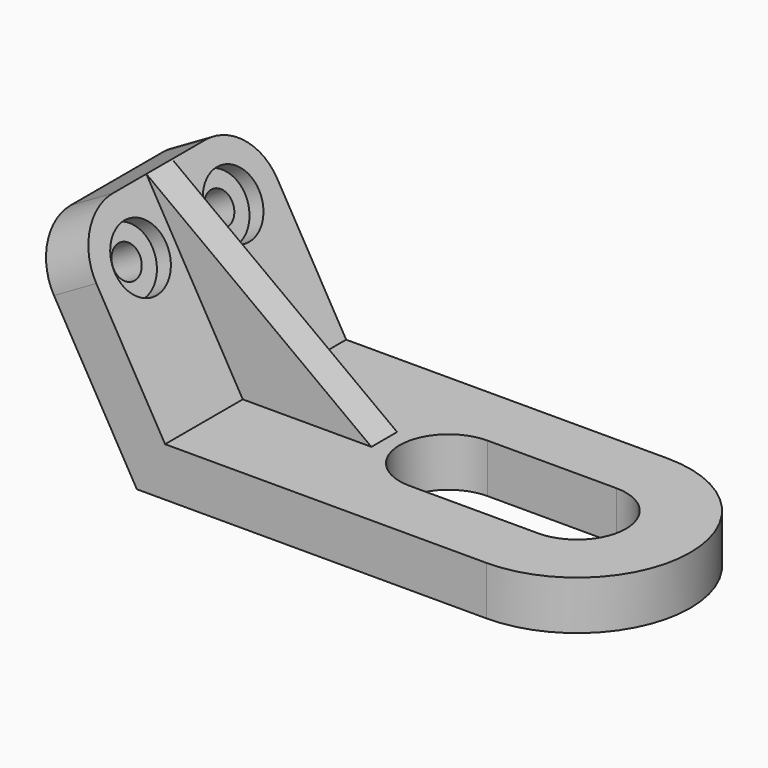
from build123d import *

# Parameters (mm, degrees)
F1_DEPTH  = 44.704
F3_DEPTH  = 9.652
F4_DEPTH  = 9.652
F8_DEPTH  = 3.175
F9_R      = 3.175
F10_DEPTH = 9.652
F9_R_2    = 6.35
F11_DEPTH = 3.175
F12_R     = 10.922


with BuildPart() as f1:
    # F0 (on Front) → F1 (new body)
    with BuildSketch(Plane.XZ):
        Polygon((-21.8362923991, 37.8215678842), (0, 0), (69.0725847982, 0), (69.0725847982, 9.652), (5.5725847982, 9.652), (-13.4774152018, 42.6475678842), align=None)
    extrude(amount=-F1_DEPTH)

    # F2 (on face) → F3 (join, through all)
    with BuildSketch(Plane.XY.offset(9.652)):
        with BuildLine():
            Line((69.0725847982, 12.7), (69.0725847982, 0))
            ThreePointArc((69.0725847982, 0), (91.4245847982, 22.352), (69.0725847982, 44.704))
            Line((69.0725847982, 44.704), (69.0725847982, 32.004))
            ThreePointArc((69.0725847982, 32.004), (78.7245847982, 22.352), (69.0725847982, 12.7))
        make_face()
    extrude(amount=-F3_DEPTH)

    # F2 (on face) → F4 (cut, through all)
    with BuildSketch(Plane.XY.offset(9.652)):
        with BuildLine():
            Line((43.6725847982, 12.7), (69.0725847982, 12.7))
            Line((69.0725847982, 12.7), (69.0725847982, 32.004))
            Line((69.0725847982, 32.004), (43.6725847982, 32.004))
            ThreePointArc((43.6725847982, 32.004), (34.0205847982, 22.352), (43.6725847982, 12.7))
        make_face()
    extrude(amount=-F4_DEPTH, mode=Mode.SUBTRACT)

    # F7 (on offset) → F8 (join, symmetric)
    with BuildSketch(Plane.XZ.offset(-22.352)):
        Polygon((30.9725847982, 9.652), (-13.4774152018, 42.6475678842), (5.5725847982, 9.652), align=None)
    extrude(amount=F8_DEPTH, both=True)

    # F9 (on face) → F10 (cut, through all)
    with BuildSketch(Plane(origin=(8.3588771973, 0, 4.826), x_dir=(0, 1, 0), z_dir=(0.8660254038, 0, 0.5))):
        with Locations((10.922, 32.7505847982)):
            Circle(F9_R)
        with BuildLine():
            ThreePointArc((30.607, 32.7505847982), (33.782, 29.5755847982), (36.957, 32.7505847982))
            Line((36.957, 32.7505847982), (33.782, 32.7505847982))
            Line((33.782, 32.7505847982), (30.607, 32.7505847982))
        make_face()
        with BuildLine():
            Line((33.782, 32.7505847982), (36.957, 32.7505847982))
            ThreePointArc((36.957, 32.7505847982), (33.782, 35.9255847982), (30.607, 32.7505847982))
            Line((30.607, 32.7505847982), (33.782, 32.7505847982))
        make_face()
    extrude(amount=-F10_DEPTH, mode=Mode.SUBTRACT)

    # F9 (on face) → F11 (cut)
    with BuildSketch(Plane(origin=(8.3588771973, 0, 4.826), x_dir=(0, 1, 0), z_dir=(0.8660254038, 0, 0.5))):
        with Locations((10.922, 32.7505847982)):
            Circle(F9_R_2)
        with Locations((10.922, 32.7505847982)):
            Circle(F9_R, mode=Mode.SUBTRACT)
        with BuildLine():
            ThreePointArc((27.432, 32.7505847982), (33.782, 26.4005847982), (40.132, 32.7505847982))
            Line((40.132, 32.7505847982), (36.957, 32.7505847982))
            ThreePointArc((36.957, 32.7505847982), (33.782, 29.5755847982), (30.607, 32.7505847982))
            Line((30.607, 32.7505847982), (27.432, 32.7505847982))
        make_face()
        with BuildLine():
            Line((36.957, 32.7505847982), (40.132, 32.7505847982))
            ThreePointArc((40.132, 32.7505847982), (33.782, 39.1005847982), (27.432, 32.7505847982))
            Line((27.432, 32.7505847982), (30.607, 32.7505847982))
            ThreePointArc((30.607, 32.7505847982), (33.782, 35.9255847982), (36.957, 32.7505847982))
        make_face()
    extrude(amount=-F11_DEPTH, mode=Mode.SUBTRACT)

    # F12
    f12_edges = [f1.edges().sort_by_distance(p)[0] for p in [
        (-17.656854, 0, 40.234568),
        (-17.656854, 44.704, 40.234568),
    ]]
    fillet(f12_edges, radius=F12_R)


solid = f1.part
